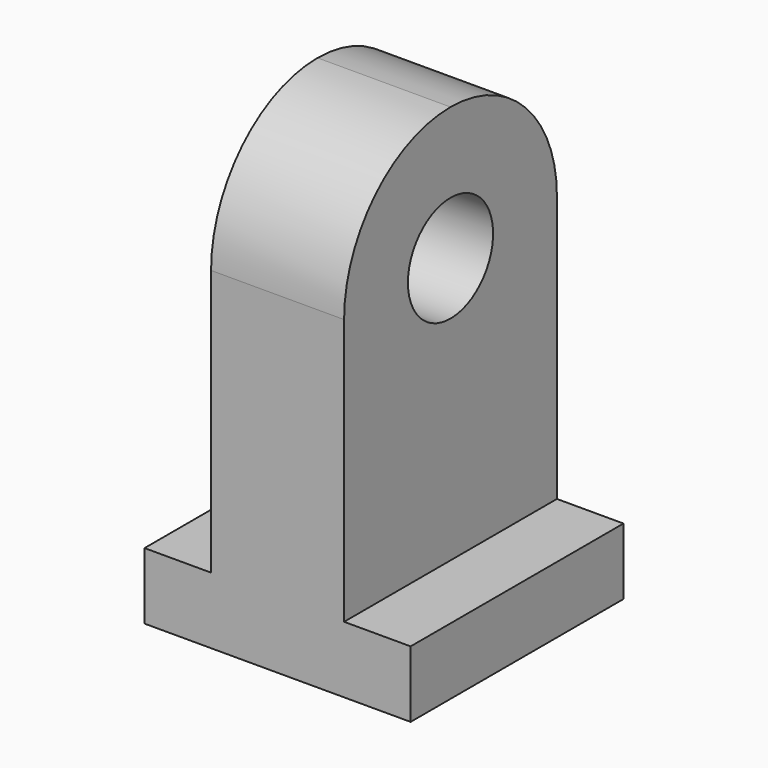
from build123d import *

# Parameters (mm, degrees)
F0_W     = 10
F0_H     = 30
F1_DEPTH = 20
F2_R     = 9.99999
F3_R     = 4
F4_DEPTH = 15.001


# Not quite as in the source:
# - a fillet or chamfer is up to 0.001 mm smaller than in the source, because OpenCascade refuses the exact size


with BuildPart() as f1:
    # F0 (on Front) → F1 (new body)
    with BuildSketch(Plane.XZ):
        with Locations((0, 20)):
            Rectangle(F0_W, F0_H)
        Polygon((-5, 5), (-10, 5), (-10, 0), (10, 0), (10, 5), (5, 5), align=None)
    extrude(amount=F1_DEPTH)

    # F2 (radius 10 in the source; OpenCascade refuses exactly that, so slightly less here)
    f2_edges = [f1.edges().sort_by_distance(p)[0] for p in [
        (0, 0, 35),
        (0, -20, 35),
    ]]
    fillet(f2_edges, radius=F2_R)

    # F3 (on face) → F4 (cut, through all)
    with BuildSketch(Plane(origin=(-5, 0, 0), x_dir=(0, -1, 0), z_dir=(-1, 0, 0))):
        with Locations((10, 25)):
            Circle(F3_R)
    extrude(amount=-F4_DEPTH, mode=Mode.SUBTRACT)


solid = f1.part
